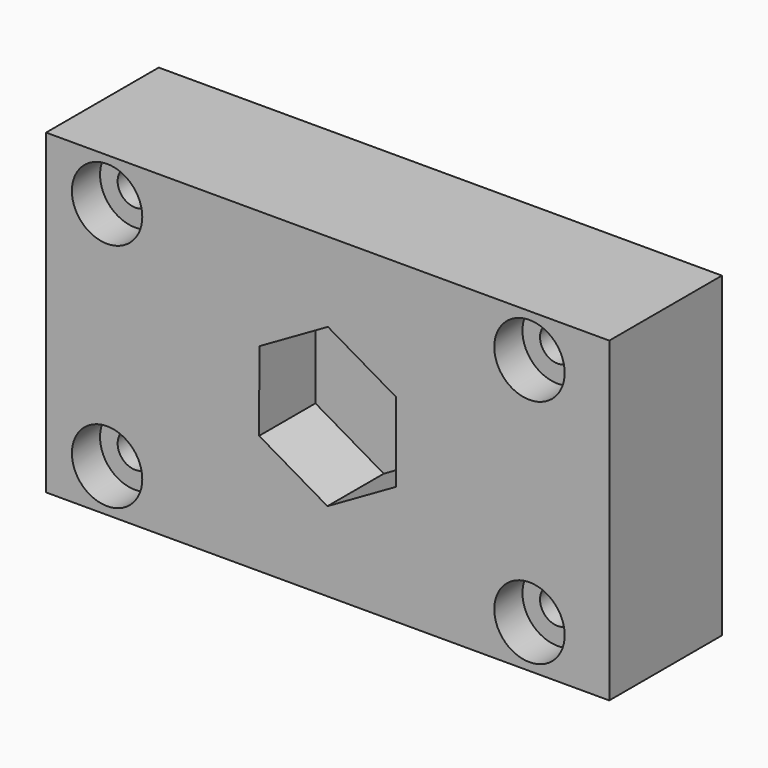
from build123d import *

# Parameters (mm, degrees)
F0_W           = 101.6
F0_H           = 57.15
F1_DEPTH       = 25.4
F3_D           = 6.35
F3_CBORE_D     = 12.7
F3_CBORE_DEPTH = 6.35
F5_DEPTH       = 12.7


with BuildPart() as f1:
    # F0 (on Front) → F1 (new body)
    with BuildSketch(Plane.XZ):
        Rectangle(F0_W, F0_H)
    extrude(amount=F1_DEPTH)

    # F3 (through all)
    with Locations(Plane.XZ.offset(25.4)):
        with Locations((36.4028997615, 20.831474103), (36.4028997615, -20.831474103), (-39.7971002385, 20.831474103), (-39.7971002385, -20.831474103)):
            CounterBoreHole(F3_D / 2, F3_CBORE_D / 2, F3_CBORE_DEPTH)

    # F4 (on face) → F5 (cut)
    with BuildSketch(Plane.XZ.offset(25.4)):
        Polygon((-0.0431249981, -14.2548758505), (12.3235221152, -7.1647852691), (12.3666471133, 7.0900905813), (0.0431249981, 14.2548758505), (-12.3235221152, 7.1647852691), (-12.3666471133, -7.0900905813), align=None)
    extrude(amount=-F5_DEPTH, mode=Mode.SUBTRACT)


solid = f1.part
